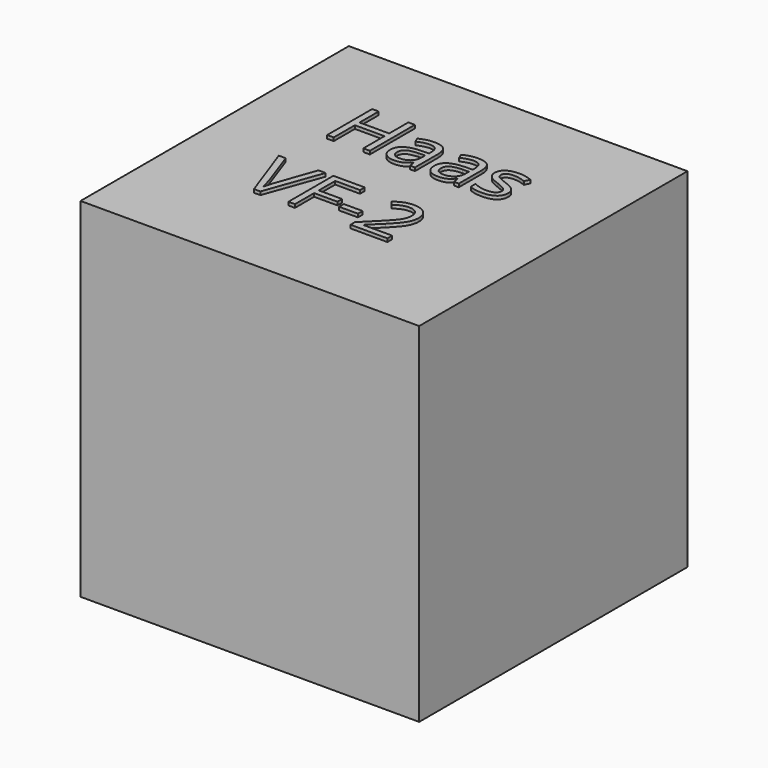
from build123d import *

# Parameters (mm, degrees)
F0_W         = 2616.2
F0_H         = 2590.8
F1_DEPTH     = 2692.4
F2_TEXT_SIZE = 608.2825776603
F3_DEPTH     = 25.4


# Not quite as in the source:
# - Text() gives the source's letters only with a copy of the font that has no kerning and outlines rounded to 1/6400 em; it was checked with that copy


with BuildPart() as f1:
    # F0 (on Top) → F1 (new body)
    with BuildSketch(Plane.XY):
        Rectangle(F0_W, F0_H)
    extrude(amount=F1_DEPTH)

    # F2 (on face) → F3 (join)
    with BuildSketch(Plane.XY.offset(2692.4)):
        with Locations((-713.496454765, 268.6477005482)):
            Text('Haas', F2_TEXT_SIZE, font='Open Sans', text_align=(TextAlign.LEFT, TextAlign.BOTTOM))
        with Locations((-713.496454765, -558.6166050699)):
            Text('VF-2', F2_TEXT_SIZE, font='Open Sans', text_align=(TextAlign.LEFT, TextAlign.BOTTOM))
    extrude(amount=F3_DEPTH)


solid = f1.part
